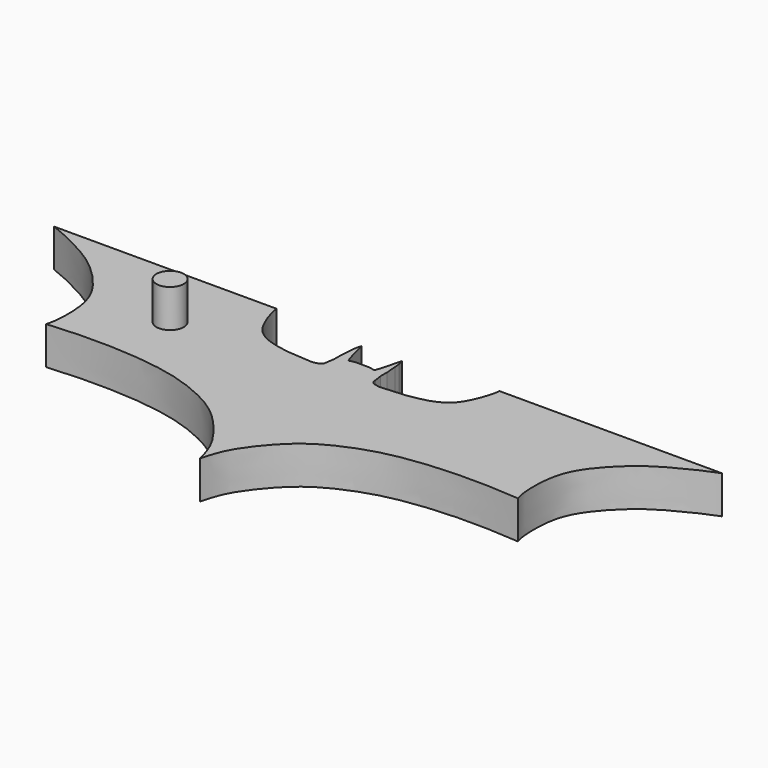
from build123d import *

# Parameters (mm, degrees)
F1_DEPTH = 25
F2_R     = 8.9966602053
F3_DEPTH = 25


with BuildPart() as f1:
    # F0 (on Top) → F1 (new body)
    with BuildSketch(Plane.XY):
        with BuildLine():
            add(Edge.make_bspline(
                [(0, 55.8526235752), (1.4280795362, 55.9029637891), (4.3012554156, 56.0042440643), (7.1458772439, 55.3181953486), (8.5766120037, 54.9731393785)],
                knots=[0, 0, 0, 0, 0.4970386764, 1, 1, 1, 1], degree=3))
            add(Edge.make_bspline(
                [(0, 55.8526235752), (-1.4280795362, 55.9029637891), (-4.3012554156, 56.0042440643), (-7.1458772439, 55.3181953486), (-8.5766120037, 54.9731393785)],
                knots=[0, 0, 0, 0, 0.4970386764, 1, 1, 1, 1], degree=3))
            add(Edge.make_bspline(
                [(-8.5766120037, 54.9731393785), (-9.6514692623, 57.7199939494), (-10.7798098483, 62.0912705565), (-12.5229449449, 68.4425182702), (-13.3537546584, 71.6931354436)],
                knots=[0, 0, 0, 0, 0.4692370062, 1, 1, 1, 1], degree=3))
            Line((-13.3537546584, 71.6931354436), (-14.3104480225, 68.1894228319))
            Line((-14.3104480225, 68.1894228319), (-14.6904686593, 64.2203330608))
            Line((-14.6904686593, 64.2203330608), (-15.2393841705, 57.2533148191))
            Line((-15.2393841705, 57.2533148191), (-15.2393841705, 51.8063676534))
            Line((-15.2393841705, 51.8063676534), (-16.0416477287, 46.5545669952))
            add(Edge.make_bspline(
                [(-16.0416477287, 46.5545669952), (-16.0782398272, 45.9712438272), (-16.1541405962, 44.7612919849), (-17.36128719, 42.9541275979), (-21.487150658, 42.106860984), (-22.7709461909, 42.1169743448), (-23.2831265938, 42.1210091502)],
                knots=[0, 0, 0, 0, 0.2160094844, 0.4480553625, 0.7797973123, 1, 1, 1, 1], degree=3))
            add(Edge.make_bspline(
                [(-23.2831265938, 42.1210091502), (-27.2965375372, 42.3088440811), (-35.3259108761, 42.6846333556), (-47.3113383189, 44.4505093957), (-57.81741508, 47.8092168889), (-66.8624396005, 55.0249311035), (-72.763514145, 71.5001102031), (-73.2202899067, 75.5655462835), (-73.3840514825, 77.0230715613)],
                knots=[0, 0, 0, 0, 0.1734744818, 0.3470592468, 0.5097817941, 0.6791962113, 0.8849865987, 1, 1, 1, 1], degree=3))
            Line((-73.3840514825, 77.0230715613), (-219.8993484104, 77.0230715613))
            add(Edge.make_bspline(
                [(-219.8993484104, 77.0230715613), (-216.7514866718, 75.7734251957), (-210.364333067, 73.237836294), (-200.8266893884, 68.423468755), (-189.669984007, 62.6285144966), (-180.5212779679, 56.1377515198), (-170.6837735136, 47.2457974455), (-162.5934600363, 37.6993260588), (-153.3213038909, 22.5624126907), (-153.1788353257, -2.3664218304), (-154.7666973105, -8.2358443771), (-155.342458745, -10.3641068946)],
                knots=[0, 0, 0, 0, 0.0982467279, 0.1993470471, 0.3080851749, 0.4119626995, 0.5229658015, 0.6311769641, 0.7614646207, 0.913506669, 1, 1, 1, 1], degree=3))
            add(Edge.make_bspline(
                [(-155.342458745, -10.3641068946), (-151.1078703147, -10.017185236), (-140.6470011893, -9.1601711182), (-110.3631366823, -8.3829172418), (-69.6209011536, -12.5152355728), (-40.4084978403, -24.8146934434), (-23.8256078227, -36.5719180218), (-4.7595753666, -59.7522314236), (-1.4611931069, -72.2254798237), (0, -77.7511657961)],
                knots=[0, 0, 0, 0, 0.1052665669, 0.2600441101, 0.443479225, 0.5997543907, 0.7273978551, 0.8792364427, 1, 1, 1, 1], degree=3))
            add(Edge.make_bspline(
                [(155.342458745, -10.3641068946), (151.1078703147, -10.017185236), (140.6470011893, -9.1601711182), (110.3631366823, -8.3829172418), (69.6209011536, -12.5152355728), (40.4084978403, -24.8146934434), (23.8256078227, -36.5719180218), (4.7595753666, -59.7522314236), (1.4611931069, -72.2254798237), (0, -77.7511657961)],
                knots=[0, 0, 0, 0, 0.1052665669, 0.2600441101, 0.443479225, 0.5997543907, 0.7273978551, 0.8792364427, 1, 1, 1, 1], degree=3))
            add(Edge.make_bspline(
                [(219.8993484104, 77.0230715613), (216.7514866718, 75.7734251957), (210.364333067, 73.237836294), (200.8266893884, 68.423468755), (189.669984007, 62.6285144966), (180.5212779679, 56.1377515198), (170.6837735136, 47.2457974455), (162.5934600363, 37.6993260588), (153.3213038909, 22.5624126907), (153.1788353257, -2.3664218304), (154.7666973105, -8.2358443771), (155.342458745, -10.3641068946)],
                knots=[0, 0, 0, 0, 0.0982467279, 0.1993470471, 0.3080851749, 0.4119626995, 0.5229658015, 0.6311769641, 0.7614646207, 0.913506669, 1, 1, 1, 1], degree=3))
            Line((219.8993484104, 77.0230715613), (73.3840514825, 77.0230715613))
            add(Edge.make_bspline(
                [(23.2831265938, 42.1210091502), (27.2965375372, 42.3088440811), (35.3259108761, 42.6846333556), (47.3113383189, 44.4505093957), (57.81741508, 47.8092168889), (66.8624396005, 55.0249311035), (72.763514145, 71.5001102031), (73.2202899067, 75.5655462835), (73.3840514825, 77.0230715613)],
                knots=[0, 0, 0, 0, 0.1734744818, 0.3470592468, 0.5097817941, 0.6791962113, 0.8849865987, 1, 1, 1, 1], degree=3))
            add(Edge.make_bspline(
                [(16.0416477287, 46.5545669952), (16.0782398272, 45.9712438272), (16.1541405962, 44.7612919849), (17.36128719, 42.9541275979), (21.487150658, 42.106860984), (22.7709461909, 42.1169743448), (23.2831265938, 42.1210091502)],
                knots=[0, 0, 0, 0, 0.2160094844, 0.4480553625, 0.7797973123, 1, 1, 1, 1], degree=3))
            Line((16.0416477287, 46.5545669952), (15.2393841705, 51.8063676534))
            Line((15.2393841705, 51.8063676534), (15.2393841705, 57.2533148191))
            Line((15.2393841705, 57.2533148191), (14.6904686593, 64.2203330608))
            Line((14.6904686593, 64.2203330608), (14.3104480225, 68.1894228319))
            Line((14.3104480225, 68.1894228319), (13.3537546584, 71.6931354436))
            add(Edge.make_bspline(
                [(8.5766120037, 54.9731393785), (9.6514692623, 57.7199939494), (10.7798098483, 62.0912705565), (12.5229449449, 68.4425182702), (13.3537546584, 71.6931354436)],
                knots=[0, 0, 0, 0, 0.4692370062, 1, 1, 1, 1], degree=3))
        make_face()
    extrude(amount=F1_DEPTH)

    # F2 (on face) → F3 (join)
    with BuildSketch(Plane.XY.offset(25)):
        with Locations((-106.9225072861, 31.2201026827)):
            Circle(F2_R)
    extrude(amount=F3_DEPTH)


solid = f1.part
